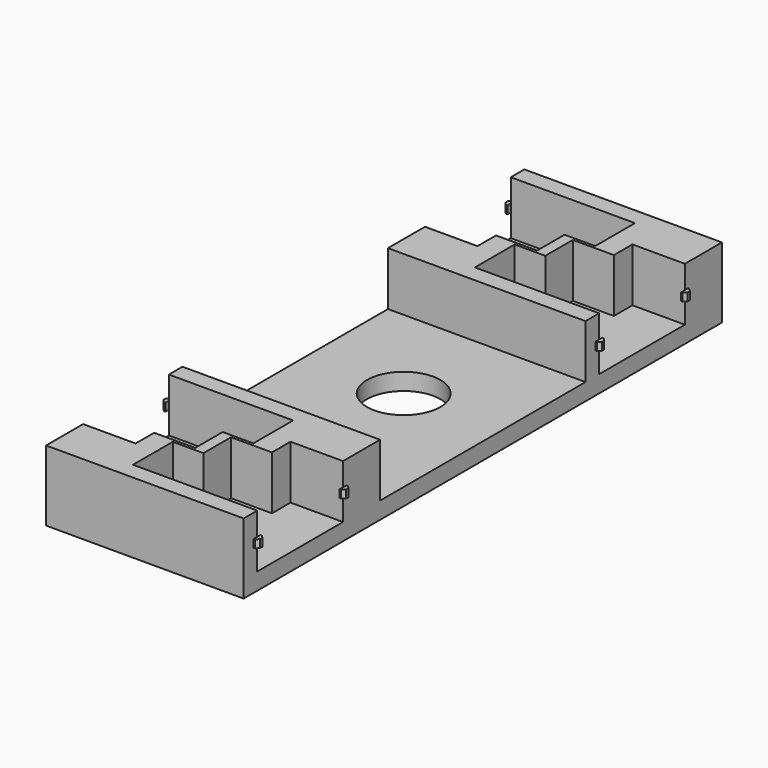
from build123d import *

# Parameters (mm, degrees)
F0_R     = 6.5
F1_DEPTH = 3
F2_DEPTH = 9.5
F3_W     = 0.6965331137
F3_H     = 1.3967012055
F3_W_2   = 0.8034668863
F3_W_3   = 0.836771971
F3_W_4   = 0.663228029
F3_W_5   = 0.7633265793
F3_W_6   = 0.7366734207
F3_W_7   = 0.7139041424
F3_W_8   = 0.7860958576
F4_DEPTH = 0.75
F5_W     = 0.7277277052
F5_H     = 1.3967012055
F5_W_2   = 0.7722722948
F5_W_3   = 0.7690980434
F5_W_4   = 0.7309019566
F5_W_5   = 0.6904412746
F5_W_6   = 0.8095587254
F5_W_7   = 0.7503486574
F5_W_8   = 0.7496513426
F6_DEPTH = 0.75
F7_SIZE  = 0.5


# Not quite as in the source:
# - ends of sketch curves that miss each other by under 0.0002 mm in the source are joined
# - a feature names something its author has since deleted; it is built from what else it names


with BuildPart() as f1:
    # F0 (on Top) → F1 (new body)
    with BuildSketch(Plane.XY):
        Polygon((7.8607099131, 16.1003852367), (-9.6392899379, 16.1003852367), (-9.6392899379, -29.3996147633), (25.3607097641, -29.3996147633), (25.3607097641, 16.1003852367), align=None)
        with Locations((7.8607099131, -2.2867515218)):
            Circle(F0_R, mode=Mode.SUBTRACT)
        Polygon((25.3607097641, -29.3996147633), (-9.6392899379, -29.3996147633), (-9.6392899379, -32.3996147633), (-6.4715547308, -32.3996147633), (12.3607100621, -32.3996147633), (25.3607097641, -32.3996147633), align=None)
        Polygon((-9.6392899379, 46.3003852367), (-9.6392899379, 43.3003852367), (-6.4715547308, 43.3003852367), (12.3607100621, 43.3003852367), (25.3607097641, 43.3003852367), (25.3607097641, 46.3003852367), align=None)
        Polygon((16.0607097641, 38.1003852367), (25.3607097641, 38.1003852367), (25.3607097641, 43.3003852367), (12.3607100621, 43.3003852367), (12.3607100621, 35.3003852367), (12.3607100621, 34.5003852367), (7.8607097641, 34.5003852367), (7.8607100621, 33.9926332235), (8.7954637781, 33.9926332235), (16.0607097641, 33.9926332235), align=None)
        Polygon((-9.6392899379, 43.3003852367), (-9.6392899379, 24.3003852367), (-0.3392899379, 24.3003852367), (-0.3392899379, 28.4081372499), (6.9259563461, 28.4081372499), (6.9259563461, 34.5003852367), (7.8607100621, 34.5003852367), (12.3607100621, 34.5003852367), (12.3607100621, 35.3003852367), (12.3607100621, 43.3003852367), (-6.4715547308, 43.3003852367), align=None)
        Polygon((3.3607097641, 27.1003852367), (3.3607097641, 19.1003852367), (22.192974557, 19.1003852367), (25.3607097641, 19.1003852367), (25.3607097641, 38.1003852367), (16.0607097641, 38.1003852367), (16.0607097641, 33.9926332235), (8.7954637781, 33.9926332235), (8.7954637781, 27.9003852367), (7.8607100621, 27.9003852367), (3.3607097641, 27.9003852367), align=None)
        Polygon((-9.6392899379, 19.1003852367), (-9.6392899379, 16.1003852367), (7.8607099131, 16.1003852367), (25.3607097641, 16.1003852367), (25.3607097641, 19.1003852367), (22.192974557, 19.1003852367), (3.3607097641, 19.1003852367), align=None)
        Polygon((-9.6392899379, 24.3003852367), (-9.6392899379, 19.1003852367), (3.3607097641, 19.1003852367), (3.3607097641, 27.1003852367), (3.3607097641, 27.9003852367), (7.8607100621, 27.9003852367), (7.8607100621, 28.4081372499), (6.9259563461, 28.4081372499), (-0.3392899379, 28.4081372499), (-0.3392899379, 24.3003852367), align=None)
        Polygon((6.9259563461, 34.5003852367), (6.9259563461, 28.4081372499), (7.8607097641, 28.4081372499), (7.8607100621, 33.9926332235), (7.8607100621, 34.5003852367), align=None)
        Polygon((7.8607100621, 28.4081372499), (7.8607100621, 27.9003852367), (8.7954637781, 27.9003852367), (8.7954637781, 33.9926332235), (7.8607097641, 33.9926332235), align=None)
        Polygon((-6.4715547308, -32.3996147633), (-9.6392899379, -32.3996147633), (-9.6392899379, -51.3996147633), (-0.3392899379, -51.3996147633), (-0.3392899379, -47.2918627501), (6.9259563461, -47.2918627501), (6.9259563461, -41.1996147633), (7.8607100621, -41.1996147633), (12.3607100621, -41.1996147633), (12.3607100621, -40.3996147633), (12.3607100621, -32.3996147633), align=None)
        Polygon((25.3607097641, -56.5996147633), (25.3607097641, -37.5996147633), (16.0607097641, -37.5996147633), (16.0607097641, -41.7073667765), (8.7954637781, -41.7073667765), (8.7954637781, -47.7996147633), (7.8607100621, -47.7996147633), (3.3607097641, -47.7996147633), (3.3607097641, -48.5996147633), (3.3607097641, -56.5996147633), (22.192974557, -56.5996147633), align=None)
        Polygon((25.3607097641, -37.5996147633), (25.3607097641, -32.3996147633), (12.3607100621, -32.3996147633), (12.3607100621, -40.3996147633), (12.3607100621, -41.1996147633), (7.8607097641, -41.1996147633), (7.8607100621, -41.7073667765), (8.7954637781, -41.7073667765), (16.0607097641, -41.7073667765), (16.0607097641, -37.5996147633), align=None)
        Polygon((-0.3392899379, -51.3996147633), (-9.6392899379, -51.3996147633), (-9.6392899379, -56.5996147633), (3.3607097641, -56.5996147633), (3.3607097641, -48.5996147633), (3.3607097641, -47.7996147633), (7.8607100621, -47.7996147633), (7.8607100621, -47.2918627501), (6.9259563461, -47.2918627501), (-0.3392899379, -47.2918627501), align=None)
        Polygon((8.7954637781, -47.7996147633), (8.7954637781, -41.7073667765), (7.8607097641, -41.7073667765), (7.8607100621, -47.2918627501), (7.8607100621, -47.7996147633), align=None)
        Polygon((6.9259563461, -41.1996147633), (6.9259563461, -47.2918627501), (7.8607097641, -47.2918627501), (7.8607100621, -41.7073667765), (7.8607100621, -41.1996147633), align=None)
        Polygon((3.3607097641, -56.5996147633), (-9.6392899379, -56.5996147633), (-9.6392899379, -59.5996147633), (25.3607097641, -59.5996147633), (25.3607097641, -56.5996147633), (22.192974557, -56.5996147633), align=None)
    extrude(amount=-F1_DEPTH)

    # F0 (on Top) → F2 (join)
    with BuildSketch(Plane.XY):
        Polygon((-9.6392899379, 19.1003852367), (-9.6392899379, 16.1003852367), (7.8607099131, 16.1003852367), (25.3607097641, 16.1003852367), (25.3607097641, 19.1003852367), (22.192974557, 19.1003852367), (3.3607097641, 19.1003852367), align=None)
        Polygon((-9.6392899379, 24.3003852367), (-9.6392899379, 19.1003852367), (3.3607097641, 19.1003852367), (3.3607097641, 27.1003852367), (3.3607097641, 27.9003852367), (7.8607100621, 27.9003852367), (7.8607100621, 28.4081372499), (6.9259563461, 28.4081372499), (-0.3392899379, 28.4081372499), (-0.3392899379, 24.3003852367), align=None)
        Polygon((-9.6392899379, 46.3003852367), (-9.6392899379, 43.3003852367), (-6.4715547308, 43.3003852367), (12.3607100621, 43.3003852367), (25.3607097641, 43.3003852367), (25.3607097641, 46.3003852367), align=None)
        Polygon((16.0607097641, 38.1003852367), (25.3607097641, 38.1003852367), (25.3607097641, 43.3003852367), (12.3607100621, 43.3003852367), (12.3607100621, 35.3003852367), (12.3607100621, 34.5003852367), (7.8607097641, 34.5003852367), (7.8607100621, 33.9926332235), (8.7954637781, 33.9926332235), (16.0607097641, 33.9926332235), align=None)
        Polygon((6.9259563461, 34.5003852367), (6.9259563461, 28.4081372499), (7.8607097641, 28.4081372499), (7.8607100621, 33.9926332235), (7.8607100621, 34.5003852367), align=None)
        Polygon((7.8607100621, 28.4081372499), (7.8607100621, 27.9003852367), (8.7954637781, 27.9003852367), (8.7954637781, 33.9926332235), (7.8607097641, 33.9926332235), align=None)
        Polygon((25.3607097641, -29.3996147633), (-9.6392899379, -29.3996147633), (-9.6392899379, -32.3996147633), (-6.4715547308, -32.3996147633), (12.3607100621, -32.3996147633), (25.3607097641, -32.3996147633), align=None)
        Polygon((25.3607097641, -37.5996147633), (25.3607097641, -32.3996147633), (12.3607100621, -32.3996147633), (12.3607100621, -40.3996147633), (12.3607100621, -41.1996147633), (7.8607097641, -41.1996147633), (7.8607100621, -41.7073667765), (8.7954637781, -41.7073667765), (16.0607097641, -41.7073667765), (16.0607097641, -37.5996147633), align=None)
        Polygon((-0.3392899379, -51.3996147633), (-9.6392899379, -51.3996147633), (-9.6392899379, -56.5996147633), (3.3607097641, -56.5996147633), (3.3607097641, -48.5996147633), (3.3607097641, -47.7996147633), (7.8607100621, -47.7996147633), (7.8607100621, -47.2918627501), (6.9259563461, -47.2918627501), (-0.3392899379, -47.2918627501), align=None)
        Polygon((8.7954637781, -47.7996147633), (8.7954637781, -41.7073667765), (7.8607097641, -41.7073667765), (7.8607100621, -47.2918627501), (7.8607100621, -47.7996147633), align=None)
        Polygon((6.9259563461, -41.1996147633), (6.9259563461, -47.2918627501), (7.8607097641, -47.2918627501), (7.8607100621, -41.7073667765), (7.8607100621, -41.1996147633), align=None)
        Polygon((3.3607097641, -56.5996147633), (-9.6392899379, -56.5996147633), (-9.6392899379, -59.5996147633), (25.3607097641, -59.5996147633), (25.3607097641, -56.5996147633), (22.192974557, -56.5996147633), align=None)
    extrude(amount=F2_DEPTH)

    # F3 (on face) → F4 (join)
    with BuildSketch(Plane.YZ.offset(25.3607097641)):
        with Locations((19.4486517936, 4.715041643)):
            Rectangle(F3_W, F3_H)
        with Locations((18.6986517936, 4.715041643)):
            Rectangle(F3_W_2, F3_H)
        with Locations((37.6819992512, 4.7070782166)):
            Rectangle(F3_W_3, F3_H)
        with Locations((38.4319992512, 4.7070782166)):
            Rectangle(F3_W_4, F3_H)
        with Locations((-37.2179514736, 4.7070782166)):
            Rectangle(F3_W_5, F3_H)
        with Locations((-37.9679514736, 4.7070782166)):
            Rectangle(F3_W_6, F3_H)
        with Locations((-56.2426626921, 4.715041643)):
            Rectangle(F3_W_7, F3_H)
        with Locations((-56.9926626921, 4.715041643)):
            Rectangle(F3_W_8, F3_H)
    extrude(amount=F4_DEPTH)

    # F5 (on face) → F6 (join)
    with BuildSketch(Plane(origin=(-9.6392899379, 0, 0), x_dir=(0, -1, 0), z_dir=(-1, 0, 0))):
        with Locations((51.7634786159, 4.7070782166)):
            Rectangle(F5_W, F5_H)
        with Locations((51.0134786159, 4.7070782166)):
            Rectangle(F5_W_2, F5_H)
        with Locations((32.784163785, 4.715041643)):
            Rectangle(F5_W_3, F5_H)
        with Locations((32.034163785, 4.715041643)):
            Rectangle(F5_W_4, F5_H)
        with Locations((-23.9551645994, 4.7070782166)):
            Rectangle(F5_W_5, F5_H)
        with Locations((-24.7051645994, 4.7070782166)):
            Rectangle(F5_W_6, F5_H)
        with Locations((-42.9252109081, 4.715041643)):
            Rectangle(F5_W_7, F5_H)
        with Locations((-43.6752109081, 4.715041643)):
            Rectangle(F5_W_8, F5_H)
    extrude(amount=F6_DEPTH)

    # F7
    f7_edges = [f1.edges().sort_by_distance(p)[0] for p in [
        (26.11071, 38.763613, 4.707078),
        (26.11071, 37.263613, 4.707078),
        (26.11071, 19.796918, 4.715042),
        (26.11071, 18.296918, 4.715042),
        (26.11071, -36.836288, 4.707078),
        (26.11071, -38.336288, 4.707078),
        (26.11071, -55.885711, 4.715042),
        (26.11071, -57.385711, 4.715042),
        (-10.38929, -52.127342, 4.707078),
        (-10.38929, -50.627342, 4.707078),
        (-10.38929, -33.168713, 4.715042),
        (-10.38929, -31.668713, 4.715042),
        (-10.38929, 23.609944, 4.707078),
        (-10.38929, 25.109944, 4.707078),
        (-10.38929, 42.550037, 4.715042),
        (-10.38929, 44.050037, 4.715042),
    ]]
    chamfer(f7_edges, length=F7_SIZE)


solid = f1.part
